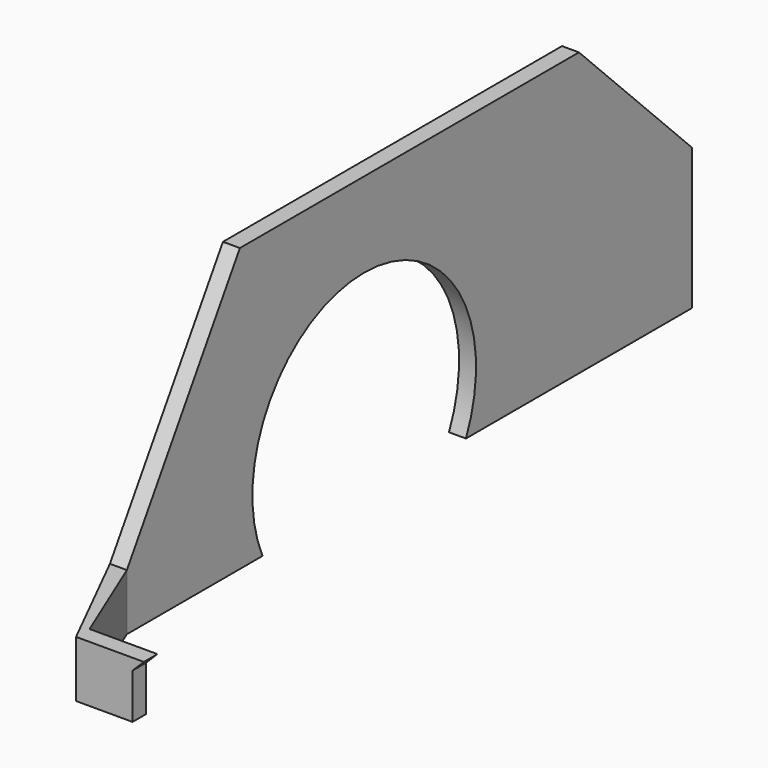
from build123d import *

# Parameters (mm, degrees)
F1_DEPTH = 10
F3_DEPTH = 3
F4_W     = 3
F4_H     = 125
F5_DEPTH = 40
F6_SIZE2 = 24.99999
F6_SIZE  = 39.99999
F7_SIZE  = 25
F9_DEPTH = 25


# Not quite as in the source:
# - a fillet or chamfer is up to 0.001 mm smaller than in the source, because OpenCascade refuses the exact size


with BuildPart() as f1:
    # F0 (on Top) → F1 (new body)
    with BuildSketch(Plane.XY):
        Polygon((0, 3), (0, 0), (10, 0), (20, 20), (20, 145), (17, 145), (17, 20), (10, 3), align=None)
    extrude(amount=F1_DEPTH)

    # F2 (on Front) → F3 (join)
    with BuildSketch(Plane.XZ):
        Polygon((0, 8), (0, 10), (-2, 10), align=None)
    extrude(amount=-F3_DEPTH)

    # F4 (on face) → F5 (join)
    with BuildSketch(Plane.XY.offset(10)):
        with Locations((18.5, 82.5)):
            Rectangle(F4_W, F4_H)
    extrude(amount=F5_DEPTH)

    # F6 (size 40 and 25 in the source; OpenCascade refuses exactly that, so slightly less here)
    f6_edges = [f1.edges().sort_by_distance(p)[0] for p in [
        (18.5, 20, 50),
    ]]
    f6_side = f1.faces().sort_by_distance((18.5, 20, 30))[0]
    chamfer(f6_edges, length=F6_SIZE, length2=F6_SIZE2, reference=f6_side)

    # F7
    f7_edges = [f1.edges().sort_by_distance(p)[0] for p in [
        (18.5, 145, 50),
    ]]
    chamfer(f7_edges, length=F7_SIZE)

    # F8 (on face) → F9 (cut)
    with BuildSketch(Plane.YZ.offset(20)):
        with BuildLine():
            Line((50, 0), (95, 0))
            ThreePointArc((95, 0), (72.5, 35), (50, 0))
        make_face()
    extrude(amount=-F9_DEPTH, mode=Mode.SUBTRACT)


with BuildPart() as f11_1:
    # F11: instance of F1
    add(f1.part.mirror(Plane.YZ.offset(-2)))


solid = f11_1.part
